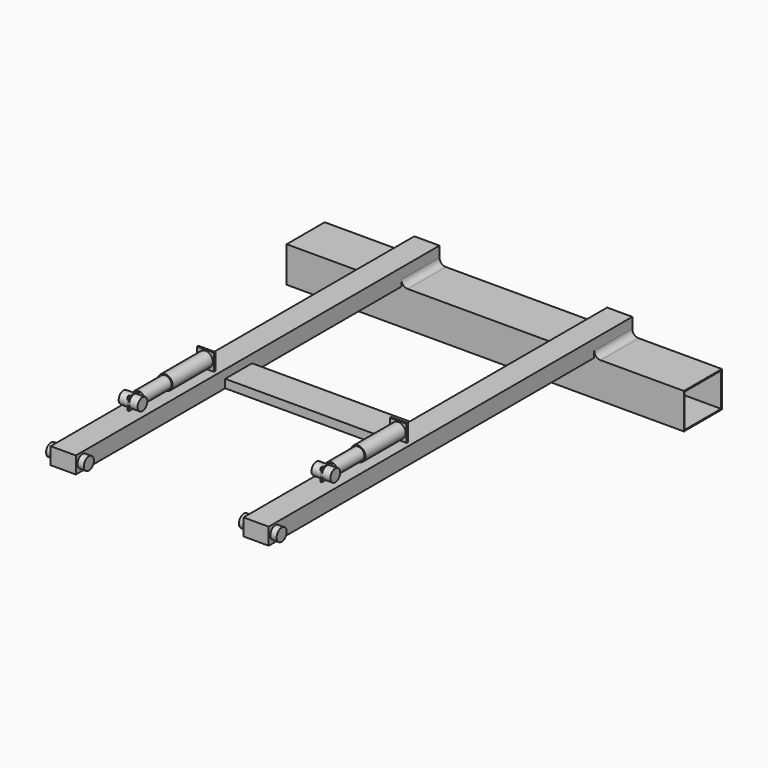
from build123d import *

# Parameters (mm, degrees)
F0_W      = 1202.4868
F0_H      = 144.018
F1_DEPTH  = 108.0135
F2_W      = 137.668
F2_H      = 101.6635
F3_DEPTH  = 1202.4868
F4_W      = 76.2
F4_H      = 144.018
F4_H_2    = 1231.9
F5_DEPTH  = 50.8
F6_R      = 19.05
F7_W      = 101.6
F7_H      = 25.4
F8_DEPTH  = 508
F9_R      = 19.05
F10_DEPTH = 19.05
F11_DEPTH = 95.25
F12_R     = 19.05
F13_DEPTH = 19.05
F14_DEPTH = 95.25
F15_W     = 50.8
F15_H     = 5.08
F16_DEPTH = 50.8
F17_R     = 22.225
F18_DEPTH = 152.4
F19_R     = 19.05
F20_DEPTH = 101.6
F22_DEPTH = 38.1
F23_R     = 18.415
F24_DEPTH = 25.4
F25_DEPTH = 31.75


with BuildPart() as f1:
    # F0 (on Top) → F1 (new body)
    with BuildSketch(Plane.XY):
        Rectangle(F0_W, F0_H)
    extrude(amount=F1_DEPTH)

    # F2 (on face) → F3 (cut)
    with BuildSketch(Plane.YZ.offset(601.2434)):
        with Locations((0, 54.00675)):
            Rectangle(F2_W, F2_H)
    extrude(amount=-F3_DEPTH, mode=Mode.SUBTRACT)

    # F4 (on face) → F5 (join)
    with BuildSketch(Plane.XY.offset(108.0135)):
        with Locations((-291.846, 0)):
            Rectangle(F4_W, F4_H)
        with Locations((291.846, 0)):
            Rectangle(F4_W, F4_H)
        with Locations((-291.846, -687.959)):
            Rectangle(F4_W, F4_H_2)
        with Locations((291.846, -687.959)):
            Rectangle(F4_W, F4_H_2)
    extrude(amount=F5_DEPTH)

    # F6
    f6_edges = [f1.edges().sort_by_distance(p)[0] for p in [
        (-253.746, 0, 108.0135),
        (-329.946, 0, 108.0135),
        (253.746, 0, 108.0135),
        (329.946, 0, 108.0135),
    ]]
    fillet(f6_edges, radius=F6_R)

    # F7 (on face) → F8 (join)
    with BuildSketch(Plane.YZ.offset(-253.746)):
        with Locations((-687.9589812279, 120.7135)):
            Rectangle(F7_W, F7_H)
    extrude(amount=F8_DEPTH)

    # F9 (on face) → F10 (join)
    with BuildSketch(Plane.YZ.offset(-253.746)):
        with Locations((-1278.509, 133.4135)):
            Circle(F9_R)
    extrude(amount=F10_DEPTH)

    # F9 (on face) → F11 (join)
    with BuildSketch(Plane.YZ.offset(-253.746)):
        with Locations((-1278.509, 133.4135)):
            Circle(F9_R)
    extrude(amount=-F11_DEPTH)

    # F12 (on face) → F13 (join)
    with BuildSketch(Plane(origin=(253.746, 0, 0), x_dir=(0, -1, 0), z_dir=(-1, 0, 0))):
        with Locations((1278.509, 133.4135)):
            Circle(F12_R)
    extrude(amount=F13_DEPTH)

    # F12 (on face) → F14 (join)
    with BuildSketch(Plane(origin=(253.746, 0, 0), x_dir=(0, -1, 0), z_dir=(-1, 0, 0))):
        with Locations((1278.509, 133.4135)):
            Circle(F12_R)
    extrude(amount=-F14_DEPTH)


with BuildPart() as f16:
    # F15 (on face) → F16 (new body)
    with BuildSketch(Plane.XY.offset(158.8135)):
        with Locations((-291.846, -763.0890947495)):
            Rectangle(F15_W, F15_H)
    extrude(amount=F16_DEPTH)

    # F17 (on face) → F18 (join)
    with BuildSketch(Plane.XZ.offset(765.6290947495)):
        with Locations((-291.846, 184.2135)):
            Circle(F17_R)
    extrude(amount=F18_DEPTH)

    # F19 (on face) → F20 (join)
    with BuildSketch(Plane.XZ.offset(918.0290947495)):
        with Locations((-291.846, 184.2135)):
            Circle(F19_R)
    extrude(amount=F20_DEPTH)

    # F21 (on face) → F22 (join)
    with BuildSketch(Plane.XZ.offset(1019.6290947495)):
        with BuildLine():
            ThreePointArc((-289.8147365776, 203.1548956431), (-290.8289176536, 203.2363295346), (-291.846, 203.2635))
            ThreePointArc((-291.846, 203.2635), (-292.8630823464, 203.2363295346), (-293.8772634224, 203.1548956431))
            Line((-293.8772634224, 203.1548956431), (-293.8772634224, 165.2721043569))
            ThreePointArc((-293.8772634224, 165.2721043569), (-292.8630823464, 165.1906704654), (-291.846, 165.1635))
            ThreePointArc((-291.846, 165.1635), (-290.8289176536, 165.1906704654), (-289.8147365776, 165.2721043569))
            Line((-289.8147365776, 165.2721043569), (-289.8147365776, 203.1548956431))
        make_face()
    extrude(amount=F22_DEPTH)

    # F23 (on face) → F24 (join)
    with BuildSketch(Plane.YZ.offset(-289.8147365776)):
        with Locations((-1038.6790947495, 184.2135)):
            Circle(F23_R)
    extrude(amount=F24_DEPTH)

    # F23 (on face) → F25 (join)
    with BuildSketch(Plane.YZ.offset(-289.8147365776)):
        with Locations((-1038.6790947495, 184.2135)):
            Circle(F23_R)
    extrude(amount=-F25_DEPTH)


with BuildPart() as f26_1:
    # F26: copy of F16
    add(f16.part.moved(Location((583.692, 0, 0))))


solid = Compound([f1.part, f16.part, f26_1.part])
